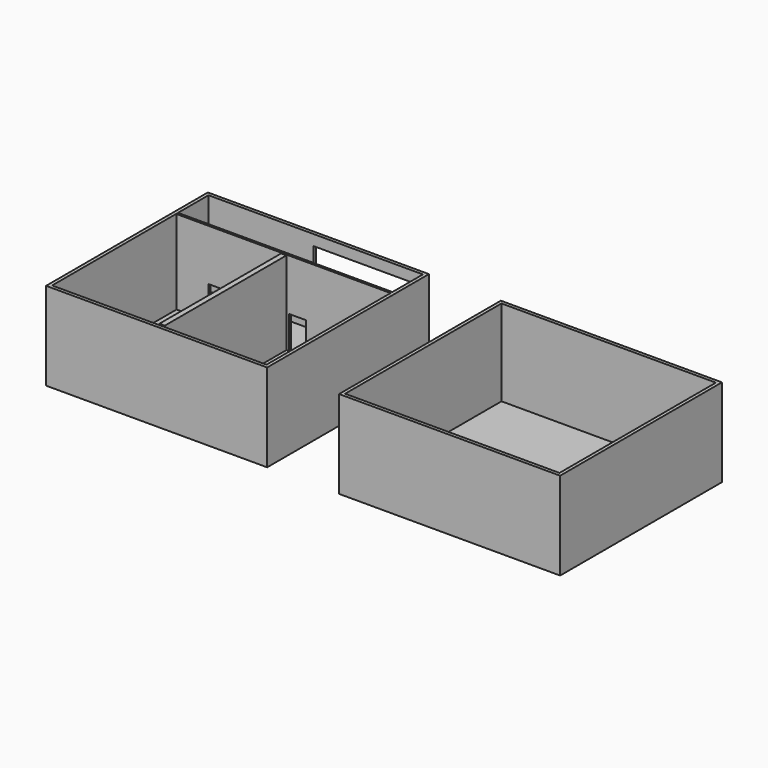
from build123d import *

# Parameters (mm, degrees)
F0_W      = 125.744625926
F0_H      = 115
F0_W_2    = 121.944625926
F0_H_2    = 111.2
F1_DEPTH  = 50
F2_DEPTH  = 2
F0_W_3    = 125.745
F0_W_4    = 121.945
F3_DEPTH  = 50
F4_DEPTH  = 1
F5_W      = 60
F5_H      = 34.5351266117
F6_DEPTH  = 12.5
F5_W_2    = 16.599290514
F5_H_2    = 25.5229242526
F8_W      = 121.944625926
F8_H      = 1.3195425272
F9_DEPTH  = 47.8
F10_W     = 10.8003032585
F10_H     = 18.6611273349
F11_DEPTH = 12.5
F10_W_2   = 9.7123030573
F10_H_2   = 18.5998911038
F13_W     = 3.026663198
F13_H     = 86.4978486359
F14_DEPTH = 47.4


# Not quite as in the source:
# - the program builds the solid bodies; features that only make, move or delete a surface that nothing else refers to are left out


with BuildPart() as f1:
    # F0 (on Top) → F1 (new body)
    with BuildSketch(Plane.XY):
        Rectangle(F0_W, F0_H)
        Rectangle(F0_W_2, F0_H_2, mode=Mode.SUBTRACT)
    extrude(amount=F1_DEPTH)

    # F0 (on Top) → F2 (join)
    with BuildSketch(Plane.XY):
        Rectangle(F0_W, F0_H)
        Rectangle(F0_W_2, F0_H_2, mode=Mode.SUBTRACT)
        Rectangle(F0_W_2, F0_H_2)
    extrude(amount=F2_DEPTH)


with BuildPart() as f3:
    # F0 (on Top) → F3 (new body)
    with BuildSketch(Plane.XY):
        with Locations((166.6439622641, 0)):
            Rectangle(F0_W_3, F0_H)
        with Locations((166.6439622641, 0)):
            Rectangle(F0_W_4, F0_H_2, mode=Mode.SUBTRACT)
    extrude(amount=F3_DEPTH)

    # F0 (on Top) → F4 (join, symmetric)
    with BuildSketch(Plane.XY):
        with Locations((166.6439622641, 0)):
            Rectangle(F0_W_4, F0_H_2)
    extrude(amount=F4_DEPTH, both=True)


with BuildPart() as f6:
    # F5 (on face) → F6 (new body, symmetric)
    with BuildSketch(Plane(origin=(0, 57.5, 0), x_dir=(-1, 0, 0), z_dir=(0, 1, 0))):
        with Locations((-28.7545890035, 26.6873809322)):
            Rectangle(F5_W, F5_H)
    extrude(amount=F6_DEPTH, both=True)


with BuildPart() as f6b:
    # F5 (on face) → F6, piece 2 (new body, symmetric)
    with BuildSketch(Plane(origin=(0, 57.5, 0), x_dir=(-1, 0, 0), z_dir=(0, 1, 0))):
        with Locations((26.2074469038, 14.7614621263)):
            Rectangle(F5_W_2, F5_H_2)
    extrude(amount=F6_DEPTH, both=True)


with BuildPart() as f1_1:
    add(f1.part)

    # F7: cut F6, F6b
    add(f6.part, mode=Mode.SUBTRACT)
    add(f6b.part, mode=Mode.SUBTRACT)

    # F8 (on face) → F9 (join)
    with BuildSketch(Plane.XY.offset(2)):
        with Locations((0, 33.5576198995)):
            Rectangle(F8_W, F8_H)
    extrude(amount=F9_DEPTH)


with BuildPart() as f11:
    # F10 (on face) → F11 (new body, symmetric)
    with BuildSketch(Plane.XZ.offset(-32.8978486359)):
        with Locations((-37.3966544867, 11.3305636675)):
            Rectangle(F10_W, F10_H)
    extrude(amount=F11_DEPTH, both=True)


with BuildPart() as f11b:
    # F10 (on face) → F11, piece 2 (new body, symmetric)
    with BuildSketch(Plane.XZ.offset(-32.8978486359)):
        with Locations((7.8935725614, 11.2999455519)):
            Rectangle(F10_W_2, F10_H_2)
    extrude(amount=F11_DEPTH, both=True)


with BuildPart() as f1_2:
    add(f1_1.part)

    # F12: cut F11, F11b
    add(f11.part, mode=Mode.SUBTRACT)
    add(f11b.part, mode=Mode.SUBTRACT)

    # F13 (on face) → F14 (join)
    with BuildSketch(Plane.XY.offset(2)):
        with Locations((-0.0097909417, -10.351075682)):
            Rectangle(F13_W, F13_H)
    extrude(amount=F14_DEPTH)


solid = Compound([f3.part, f1_2.part])
